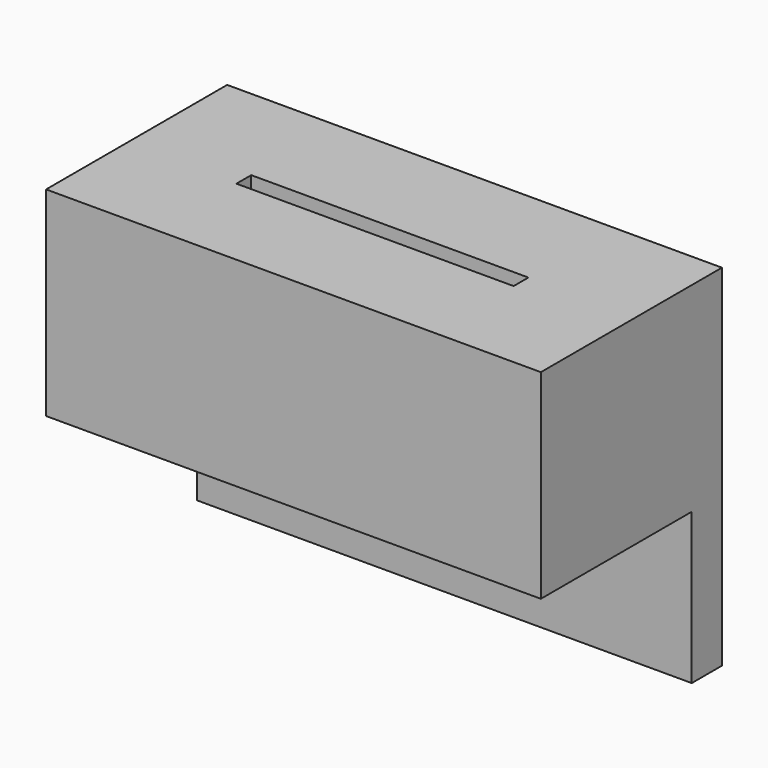
from build123d import *

# Parameters (mm, degrees)
F1_DEPTH = 38.1
F2_W     = 83.2868572325
F2_H     = 33.5878157057
F2_H_2   = 25.4
F3_DEPTH = 6.35
F4_W     = 46.6631539166
F4_H     = 3.1104013324
F5_DEPTH = 25.4


# Not quite as in the source:
# - a feature names something its author has since deleted; it is built from what else it names


with BuildPart() as f1:
    # F0 (on Front) → F1 (new body)
    with BuildSketch(Plane.XZ):
        Polygon((53.1807057559, 35.5675853789), (-30.1061514765, 35.5675853789), (-30.1061514765, 1.9797696732), (-19.1832855344, 1.9797696732), (-9.4892410561, 1.9797696732), (53.1807057559, 1.9797696732), align=None)
    extrude(amount=-F1_DEPTH)

    # F2 (on face) → F3 (join)
    with BuildSketch(Plane(origin=(0, 38.1, 0), x_dir=(-1, 0, 0), z_dir=(0, 1, 0))):
        with Locations((-11.5372771397, 18.773677526)):
            Rectangle(F2_W, F2_H)
        with Locations((-11.5372771397, -10.7202303268)):
            Rectangle(F2_W, F2_H_2)
    extrude(amount=-F3_DEPTH)

    # F4 (on face) → F5 (cut)
    with BuildSketch(Plane.XY.offset(35.5675853789)):
        with Locations((11.7438416928, 18.4589158744)):
            Rectangle(F4_W, F4_H)
    extrude(amount=-F5_DEPTH, mode=Mode.SUBTRACT)


solid = f1.part
